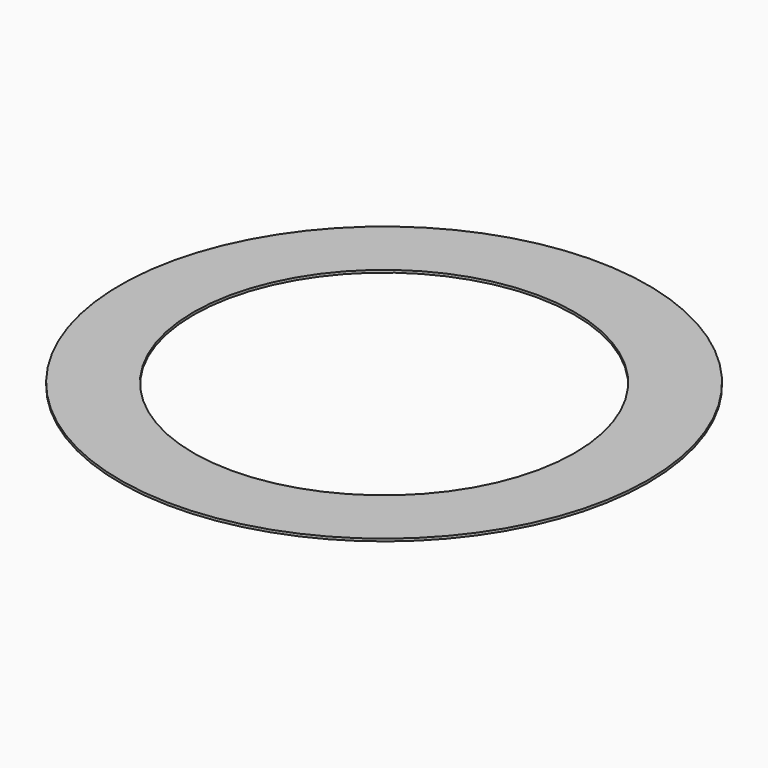
from build123d import *

# Parameters (mm, degrees)
F0_R     = 457.2
F0_R_2   = 330.2
F1_DEPTH = 4.2333333333


# Not quite as in the source:
# - a length typed as a fraction of an inch, garbled in the dataset ("3 / 203.2 mm" for 3/8 in), is restored


with BuildPart() as f1:
    # F0 (on Top) → F1 (new body)
    with BuildSketch(Plane.XY):
        Circle(F0_R)
        Circle(F0_R_2, mode=Mode.SUBTRACT)
    extrude(amount=F1_DEPTH)


solid = f1.part
